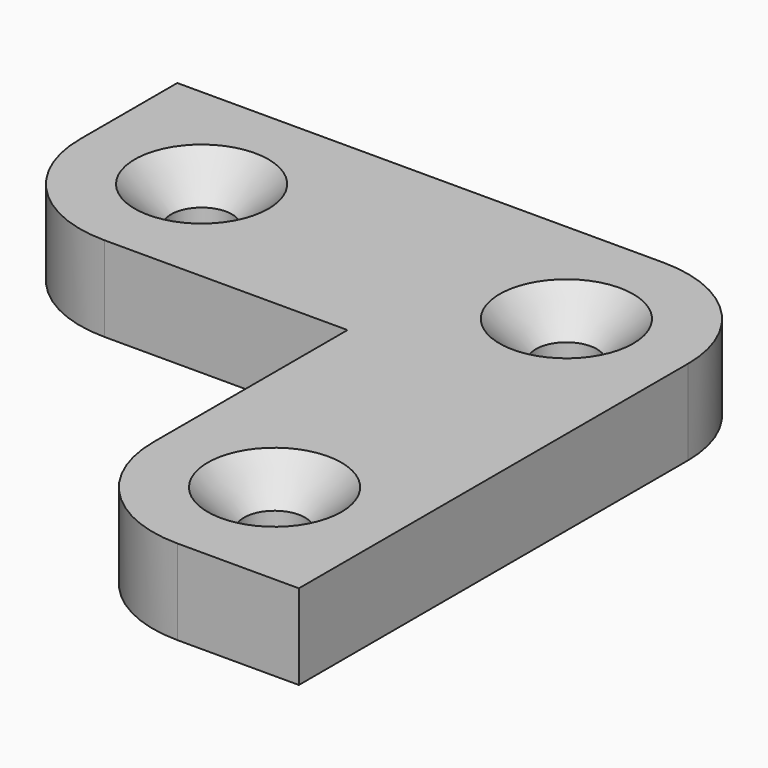
from build123d import *

# Parameters (mm, degrees)
F0_R     = 2.5
F1_DEPTH = 7
F2_R     = 10
F3_SIZE  = 3


# Not quite as in the source:
# - a feature names something its author has since deleted; it is built from what else it names


with BuildPart() as f1:
    # F0 (on Top) → F1 (new body)
    with BuildSketch(Plane.XY):
        Polygon((0, -50), (0, 0), (-50, 0), (-50, -20), (-20, -20), (-20, -50), align=None)
        with Locations((-10, -40)):
            Circle(F0_R, mode=Mode.SUBTRACT)
        with Locations((-40, -10)):
            Circle(F0_R, mode=Mode.SUBTRACT)
        with Locations((-10, -10)):
            Circle(F0_R, mode=Mode.SUBTRACT)
    extrude(amount=F1_DEPTH)

    # F2
    f2_edges = [f1.edges().sort_by_distance(p)[0] for p in [
        (0, 0, 3.5),
        (-20, -50, 3.5),
        (-50, -20, 3.5),
    ]]
    fillet(f2_edges, radius=F2_R)

    # F3
    f3_edges = [f1.edges().sort_by_distance(p)[0] for p in [
        (-42.5, -10, 7),
        (-12.5, -40, 7),
        (-12.5, -10, 7),
    ]]
    chamfer(f3_edges, length=F3_SIZE)


solid = f1.part
